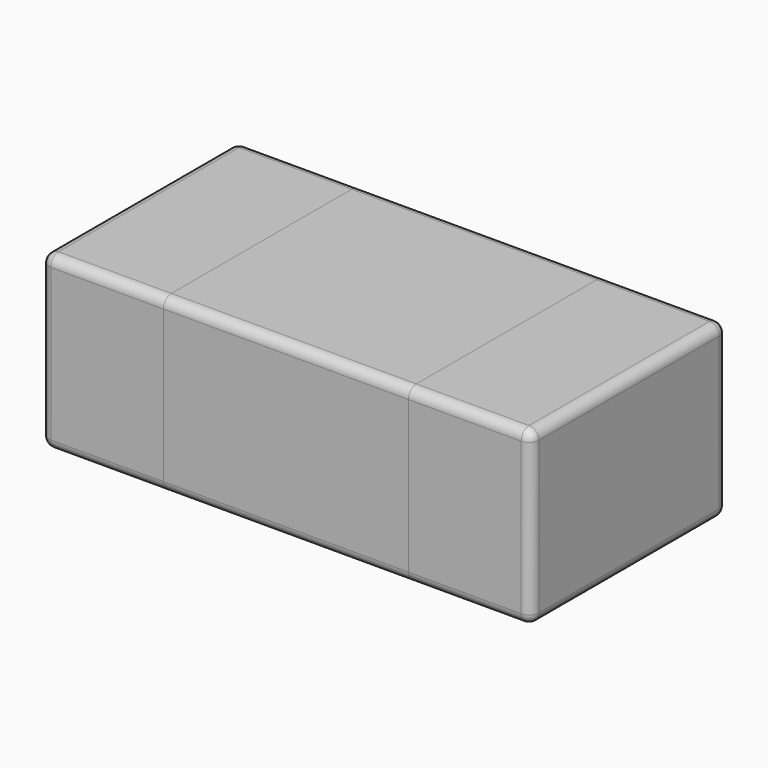
from build123d import *

# Parameters (mm, degrees)
F2_W     = 0.5
F2_H     = 0.5
F3_DEPTH = 0.33
F2_W_2   = 0.25
F4_DEPTH = 0.35
F5_DEPTH = 0.35
F6_DEPTH = 0.02
F7_R     = 0.01999
F7_2_R   = 0.01999
F7_3_R   = 0.01999
F7_4_R   = 0.01999


# Not quite as in the source:
# - a fillet or chamfer is up to 0.001 mm smaller than in the source, because OpenCascade refuses the exact size


with BuildPart() as f3:
    # F2 (on Top) → F3 (new body)
    with BuildSketch(Plane.XY):
        Rectangle(F2_W, F2_H)
    extrude(amount=F3_DEPTH)


with BuildPart() as f4:
    # F2 (on Top) → F4 (new body)
    with BuildSketch(Plane.XY):
        with Locations((-0.375, 0)):
            Rectangle(F2_W_2, F2_H)
    extrude(amount=F4_DEPTH)

    # F7 (radius 0.02 in the source; OpenCascade refuses exactly that, so slightly less here)
    f7_edges = [f4.edges().sort_by_distance(p)[0] for p in [
        (-0.375, -0.25, 0.35),
        (-0.5, 0.25, 0.175),
        (-0.5, -0.25, 0.175),
        (-0.5, 0, 0),
        (-0.5, 0, 0.35),
        (-0.375, 0.25, 0.35),
        (-0.375, 0.25, 0),
        (-0.375, -0.25, 0),
    ]]
    fillet(f7_edges, radius=F7_R)


with BuildPart() as f5:
    # F2 (on Top) → F5 (new body)
    with BuildSketch(Plane.XY):
        with Locations((0.375, 0)):
            Rectangle(F2_W_2, F2_H)
    extrude(amount=F5_DEPTH)

    # F7#2 (radius 0.02 in the source; OpenCascade refuses exactly that, so slightly less here)
    f7_2_edges = [f5.edges().sort_by_distance(p)[0] for p in [
        (0.375, -0.25, 0.35),
        (0.5, -0.25, 0.175),
        (0.5, 0.25, 0.175),
        (0.5, 0, 0),
        (0.5, 0, 0.35),
        (0.375, 0.25, 0.35),
        (0.375, 0.25, 0),
        (0.375, -0.25, 0),
    ]]
    fillet(f7_2_edges, radius=F7_2_R)


with BuildPart() as f6:
    # F6 (new): a face of the model
    f6_faces = [f3.part.faces().sort_by_distance(p)[0] for p in [
        (0, 0, 0.33),
    ]]
    extrude(f6_faces, amount=F6_DEPTH)

    # F7#4 (radius 0.02 in the source; OpenCascade refuses exactly that, so slightly less here)
    f7_4_edges = [f6.edges().sort_by_distance(p)[0] for p in [
        (0, -0.25, 0.35),
        (0, 0.25, 0.35),
    ]]
    fillet(f7_4_edges, radius=F7_4_R)


with BuildPart() as f3_1:
    add(f3.part)

    # F7#3 (radius 0.02 in the source; OpenCascade refuses exactly that, so slightly less here)
    f7_3_edges = [f3_1.edges().sort_by_distance(p)[0] for p in [
        (0, 0.25, 0),
        (0, -0.25, 0),
    ]]
    fillet(f7_3_edges, radius=F7_3_R)


solid = Compound([f4.part, f5.part, f6.part, f3_1.part])
